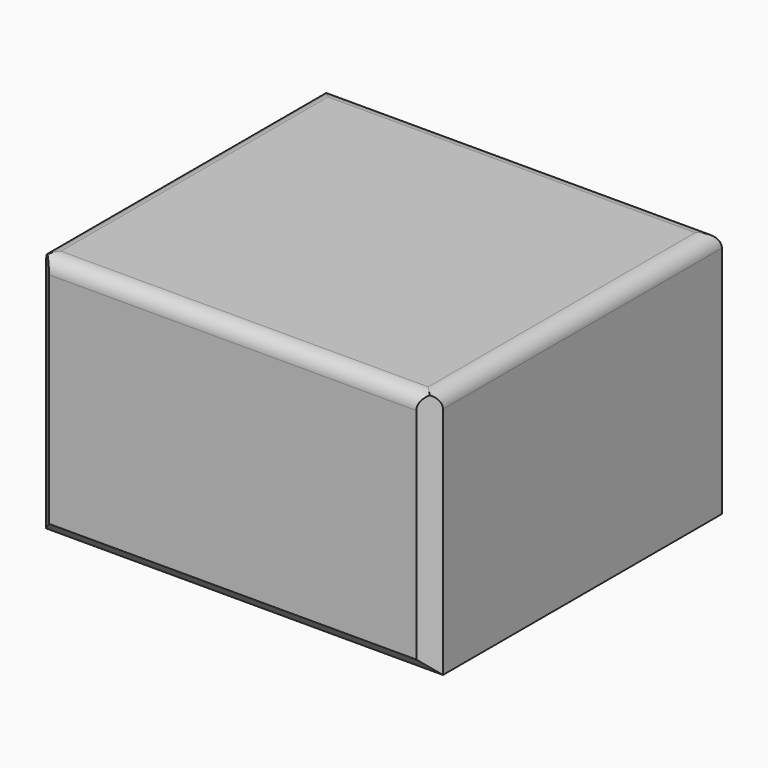
from build123d import *

# Parameters (mm, degrees)
F1_DEPTH    = 124.714
F2_R        = 5.08
F3_T1_DEPTH = 106.4324408115
F3_T3_DEPTH = 162.3159941245


# Not quite as in the source:
# - a fillet or chamfer that OpenCascade refuses, or shapes differently, is made with other operations: its cross-section is extruded or revolved along the edge and cut away or added


with BuildPart() as f1:
    # F0 (on Front) → F1 (new body)
    with BuildSketch(Plane.XZ):
        Polygon((-27.0380023867, 36.5847535431), (-68.4493109584, 36.5847535431), (-68.4493109584, -48.7993881106), (67.7383840084, -48.7993881106), (67.7383840084, 36.5847535431), (0, 36.5847535431), align=None)
    extrude(amount=F1_DEPTH)

    # F2
    f2_edges = [f1.edges().sort_by_distance(p)[0] for p in [
        (-68.449311, -62.357, 36.584754),
        (-0.355463, 0, 36.584754),
        (67.738384, -62.357, 36.584754),
        (-0.355463, -124.714, 36.584754),
    ]]
    fillet(f2_edges, radius=F2_R)

    # F3: chamfer of 5.08 on 4 edges, made by hand

    # F3_s2 → F3_t1 (cut)
    with BuildSketch(Plane.XY.offset(-61.8635376895)):
        Polygon((-68.4493109584, -119.634), (-63.3693109584, -124.714), (-68.4493109584, -124.714), align=None)
        Polygon((62.6583840084, -124.714), (67.7383840084, -119.634), (67.7383840084, -124.714), align=None)
    extrude(amount=F3_T1_DEPTH, mode=Mode.SUBTRACT)

    # F3_s4 → F3_t3 (cut)
    with BuildSketch(Plane.YZ.offset(-81.5134605373)):
        Polygon((-124.714, -43.7193881106), (-119.634, -48.7993881106), (-124.714, -48.7993881106), align=None)
    extrude(amount=F3_T3_DEPTH, mode=Mode.SUBTRACT)


solid = f1.part
